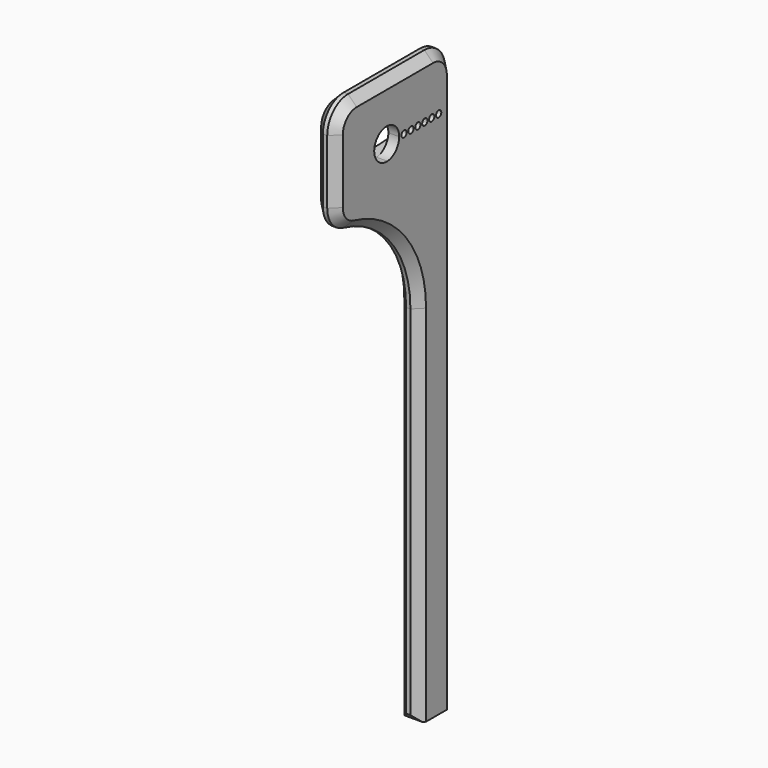
from build123d import *

# Parameters (mm, degrees)
F0_W        = 24
F0_H        = 26
F1_DEPTH    = 5
F2_T1_DEPTH = 5
F3_SIZE     = 1.5
F4_R        = 6
F5_SIZE     = 2
F6_R        = 0.75
F7_DEPTH    = 5
F8_DEPTH    = 2.5


# Not quite as in the source:
# - a fillet or chamfer that OpenCascade refuses, or shapes differently, is made with other operations: its cross-section is extruded or revolved along the edge and cut away or added


with BuildPart() as f1:
    # F0 (on Right) → F1 (new body)
    with BuildSketch(Plane.YZ):
        Rectangle(F0_W, F0_H)
        Polygon((22, 13), (12, 13), (12, -13), (12, -122), (22, -122), align=None)
    extrude(amount=F1_DEPTH)

    # F2: fillet of radius 25 on 1 edges, made by hand

    # F2_s2 → F2_t1 (join)
    with BuildSketch(Plane.YZ):
        with BuildLine():
            ThreePointArc((-12, -13), (5.0277563773, -20.6594839179), (12, -37.9799919936))
            Line((12, -37.9799919936), (12, -13))
            Line((12, -13), (-12, -13))
        make_face()
    extrude(amount=F2_T1_DEPTH)

    # F3
    f3_edges = [f1.edges().sort_by_distance(p)[0] for p in [
        (2.5, 12, -122),
        (2.5, 22, -122),
    ]]
    chamfer(f3_edges, length=F3_SIZE)

    # F4
    f4_edges = [f1.edges().sort_by_distance(p)[0] for p in [
        (2.5, -12, -13),
        (2.5, -12, 13),
        (2.5, 22, 13),
    ]]
    fillet(f4_edges, radius=F4_R)

    # F5
    f5_edges = [f1.edges().sort_by_distance(p)[0] for p in [
        (5, 22, -56.75),
        (0, 22, -56.75),
        (0, 6.572034, -22.425717),
        (0, -10.697288, -11.51368),
        (0, 12, -79.239996),
        (0, -12, -0.390327),
        (0, -10.242641, 11.242641),
        (0, 5, 13),
        (0, 20.242641, 11.242641),
        (5, 6.572034, -22.425717),
        (5, -10.697288, -11.51368),
        (5, 12, -79.239996),
        (5, -12, -0.390327),
        (5, -10.242641, 11.242641),
        (5, 5, 13),
        (5, 20.242641, 11.242641),
    ]]
    chamfer(f5_edges, length=F5_SIZE)

    # F6 (on face) → F7 (cut)
    with BuildSketch(Plane(origin=(0, 0, 0), x_dir=(0, -1, 0), z_dir=(-1, 0, 0))):
        with BuildLine():
            ThreePointArc((-2.8632404181, 3.5936789679), (-5.2698917444, 2.469041767), (-6.25, 0))
            ThreePointArc((-6.25, 0), (-5.2698917444, -2.469041767), (-2.8632404181, -3.5936789679))
            ThreePointArc((-2.8632404181, -3.5936789679), (-0.180958233, -2.6198917444), (0.95, 0))
            ThreePointArc((0.95, 0), (-0.180958233, 2.6198917444), (-2.8632404181, 3.5936789679))
        make_face()
        with BuildLine():
            ThreePointArc((-5.25, 0), (-2.65, 2.6), (-0.05, 0))
            ThreePointArc((-0.05, 0), (-2.65, -2.6), (-5.25, 0))
        make_face(mode=Mode.SUBTRACT)
        with BuildLine():
            ThreePointArc((-5.25, 0), (-2.65, -2.6), (-0.05, 0))
            ThreePointArc((-0.05, 0), (-2.65, 2.6), (-5.25, 0))
        make_face()
        with Locations((-17.65, 0)):
            Circle(F6_R)
        with BuildLine():
            Line((-16.4, 0), (-14.9, 0))
            ThreePointArc((-14.9, 0), (-15.65, 0.75), (-16.4, 0))
        make_face()
        with BuildLine():
            ThreePointArc((-16.4, 0), (-15.65, -0.75), (-14.9, 0))
            Line((-14.9, 0), (-16.4, 0))
        make_face()
        with BuildLine():
            ThreePointArc((-10.9, 0), (-11.65, 0.75), (-12.4, 0))
            Line((-12.4, 0), (-10.9, 0))
        make_face()
        with BuildLine():
            Line((-10.9, 0), (-12.4, 0))
            ThreePointArc((-12.4, 0), (-11.65, -0.75), (-10.9, 0))
        make_face()
        with BuildLine():
            ThreePointArc((-10.4, 0), (-9.65, -0.75), (-8.9, 0))
            Line((-8.9, 0), (-10.4, 0))
        make_face()
        with BuildLine():
            Line((-10.4, 0), (-8.9, 0))
            ThreePointArc((-8.9, 0), (-9.65, 0.75), (-10.4, 0))
        make_face()
        with BuildLine():
            Line((-8.4, 0), (-6.9, 0))
            ThreePointArc((-6.9, 0), (-7.65, 0.75), (-8.4, 0))
        make_face()
        with BuildLine():
            ThreePointArc((-8.4, 0), (-7.65, -0.75), (-6.9, 0))
            Line((-6.9, 0), (-8.4, 0))
        make_face()
        with BuildLine():
            ThreePointArc((-12.9, 0), (-13.4380659424, 0.719433079), (-14.2802238806, 0.406592991))
            ThreePointArc((-14.2802238806, 0.406592991), (-14.2575663793, 0.2038573909), (-14.25, 0))
            Line((-14.25, 0), (-12.9, 0))
        make_face()
        with BuildLine():
            ThreePointArc((-14.25, 0), (-14.2575663793, -0.2038573909), (-14.2802238806, -0.406592991))
            ThreePointArc((-14.2802238806, -0.406592991), (-13.4380659424, -0.719433079), (-12.9, 0))
            Line((-12.9, 0), (-14.25, 0))
        make_face()
        with BuildLine():
            ThreePointArc((-14.4, 0), (-14.369433079, -0.2119340576), (-14.2802238806, -0.406592991))
            ThreePointArc((-14.2802238806, -0.406592991), (-14.2575663793, -0.2038573909), (-14.25, 0))
            Line((-14.25, 0), (-14.4, 0))
        make_face()
        with BuildLine():
            ThreePointArc((-14.25, 0), (-14.2575663793, 0.2038573909), (-14.2802238806, 0.406592991))
            ThreePointArc((-14.2802238806, 0.406592991), (-14.369433079, 0.2119340576), (-14.4, 0))
            Line((-14.4, 0), (-14.25, 0))
        make_face()
    extrude(amount=-F7_DEPTH, mode=Mode.SUBTRACT)

    # F6 (on face) → F8 (cut)
    with BuildSketch(Plane(origin=(0, 0, 0), x_dir=(0, -1, 0), z_dir=(-1, 0, 0))):
        with BuildLine():
            ThreePointArc((-2.8632404181, -3.5936789679), (-5.2698917444, -2.469041767), (-6.25, 0))
            Line((-6.25, 0), (-6.9, 0))
            ThreePointArc((-6.9, 0), (-7.65, -0.75), (-8.4, 0))
            Line((-8.4, 0), (-8.9, 0))
            ThreePointArc((-8.9, 0), (-9.65, -0.75), (-10.4, 0))
            Line((-10.4, 0), (-10.9, 0))
            ThreePointArc((-10.9, 0), (-11.65, -0.75), (-12.4, 0))
            Line((-12.4, 0), (-12.9, 0))
            ThreePointArc((-12.9, 0), (-13.4380659424, -0.719433079), (-14.2802238806, -0.406592991))
            ThreePointArc((-14.2802238806, -0.406592991), (-15.2674725396, -2.1356143376), (-17.1628919861, -2.7451714338))
            Line((-17.1628919861, -2.7451714338), (-2.8632404181, -3.5936789679))
        make_face()
        with BuildLine():
            ThreePointArc((-14.2802238806, 0.406592991), (-15.2674725396, 2.1356143376), (-17.1628919861, 2.7451714338))
            ThreePointArc((-17.1628919861, 2.7451714338), (-19.75, 0), (-17.1628919861, -2.7451714338))
            ThreePointArc((-17.1628919861, -2.7451714338), (-15.2674725396, -2.1356143376), (-14.2802238806, -0.406592991))
            ThreePointArc((-14.2802238806, -0.406592991), (-14.369433079, -0.2119340576), (-14.4, 0))
            ThreePointArc((-14.4, 0), (-14.369433079, 0.2119340576), (-14.2802238806, 0.406592991))
        make_face()
        with Locations((-17.65, 0)):
            Circle(F6_R, mode=Mode.SUBTRACT)
        with BuildLine():
            ThreePointArc((-16.4, 0), (-15.65, 0.75), (-14.9, 0))
            ThreePointArc((-14.9, 0), (-15.65, -0.75), (-16.4, 0))
        make_face(mode=Mode.SUBTRACT)
        with BuildLine():
            Line((-6.9, 0), (-6.25, 0))
            ThreePointArc((-6.25, 0), (-5.2698917444, 2.469041767), (-2.8632404181, 3.5936789679))
            Line((-2.8632404181, 3.5936789679), (-17.1628919861, 2.7451714338))
            ThreePointArc((-17.1628919861, 2.7451714338), (-15.2674725396, 2.1356143376), (-14.2802238806, 0.406592991))
            ThreePointArc((-14.2802238806, 0.406592991), (-13.4380659424, 0.719433079), (-12.9, 0))
            Line((-12.9, 0), (-12.4, 0))
            ThreePointArc((-12.4, 0), (-11.65, 0.75), (-10.9, 0))
            Line((-10.9, 0), (-10.4, 0))
            ThreePointArc((-10.4, 0), (-9.65, 0.75), (-8.9, 0))
            Line((-8.9, 0), (-8.4, 0))
            ThreePointArc((-8.4, 0), (-7.65, 0.75), (-6.9, 0))
        make_face()
    extrude(amount=-F8_DEPTH, mode=Mode.SUBTRACT)


solid = f1.part
